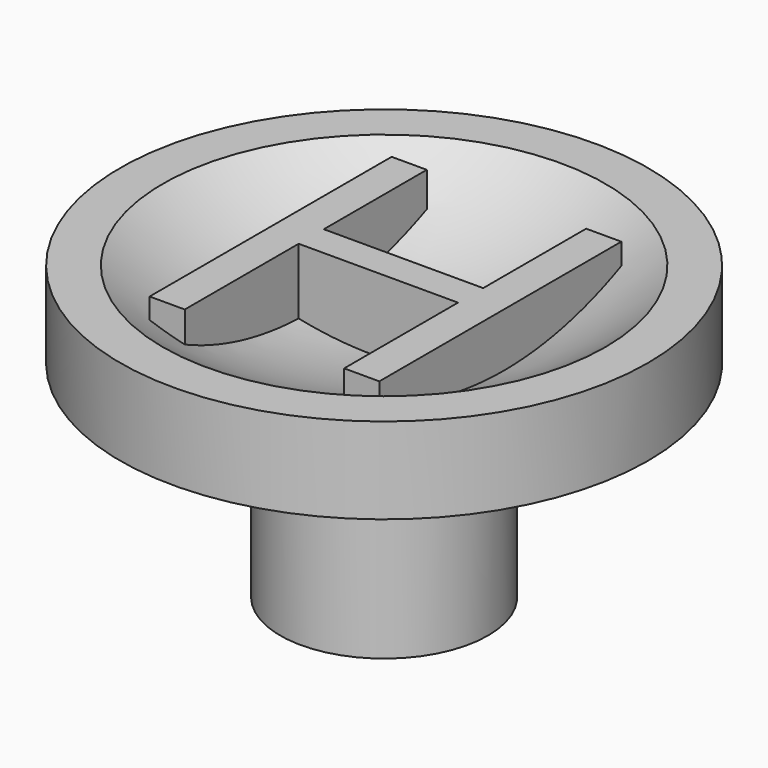
from build123d import *

# Parameters (mm, degrees)
F2_TEXT_SIZE = 16.0527208613
F3_DEPTH     = 4.064
F4_W         = 36.596095445
F4_H         = 4.7990862535
F5_DEPTH     = 12.7
F6_SIZE      = 1.27
F7_R         = 14.7196181522
F7_R_2       = 5.842
F8_DEPTH     = 0.8
F9_SIZE      = 1.016


# Not quite as in the source:
# - Text() gives the source's letters only with a copy of the font that has no kerning and outlines rounded to 1/6400 em; it was checked with that copy


with BuildPart() as f1:
    # F0 (on Front) → F1 (revolve)
    with BuildSketch(Plane.XZ):
        with BuildLine():
            Line((0, 0), (2.6757909362, 0))
            Line((2.6757909362, 0), (2.6757909362, -3.438))
            ThreePointArc((2.6757909362, -3.438), (2.2947909362, -3.819), (2.6757909362, -4.2))
            Line((2.6757909362, -4.2), (2.6757909362, -7))
            Line((2.6757909362, -7), (3.937, -7))
            Line((3.937, -7), (3.937, 0))
            Line((3.937, 0), (10, 0))
            Line((10, 0), (10, 5.4849551513))
            ThreePointArc((10, 5.4849551513), (5.4259986852, 2.3667937844), (0, 1.27))
            Line((0, 1.27), (0, 0))
        make_face()
    revolve(axis=Axis((0, 0, 0.635), (0, 0, -1)))

    # F2 (on Top) → F3 (join)
    with BuildSketch(Plane.XY):
        with Locations((-5.7483571582, -5.8876438998)):
            Text('H', F2_TEXT_SIZE, font='Open Sans', text_align=(TextAlign.LEFT, TextAlign.BOTTOM))
    extrude(amount=F3_DEPTH)

    # F4 (on Right) → F5 (cut, symmetric)
    with BuildSketch(Plane.YZ):
        with Locations((1.1354844319, 6.4635431267)):
            Rectangle(F4_W, F4_H)
    extrude(amount=F5_DEPTH, both=True, mode=Mode.SUBTRACT)

    # F6
    f6_edges = [f1.edges().sort_by_distance(p)[0] for p in [
        (-2.675791, 0, 0),
    ]]
    chamfer(f6_edges, length=F6_SIZE)

    # F7 (on face) → F8 (cut)
    with BuildSketch(Plane(origin=(0, 0, 0), x_dir=(1, 0, 0), z_dir=(0, 0, -1))):
        Circle(F7_R)
        Circle(F7_R_2, mode=Mode.SUBTRACT)
    extrude(amount=-F8_DEPTH, mode=Mode.SUBTRACT)

    # F9
    f9_edges = [f1.edges().sort_by_distance(p)[0] for p in [
        (-2.675791, 0, -7),
    ]]
    chamfer(f9_edges, length=F9_SIZE)


solid = f1.part
